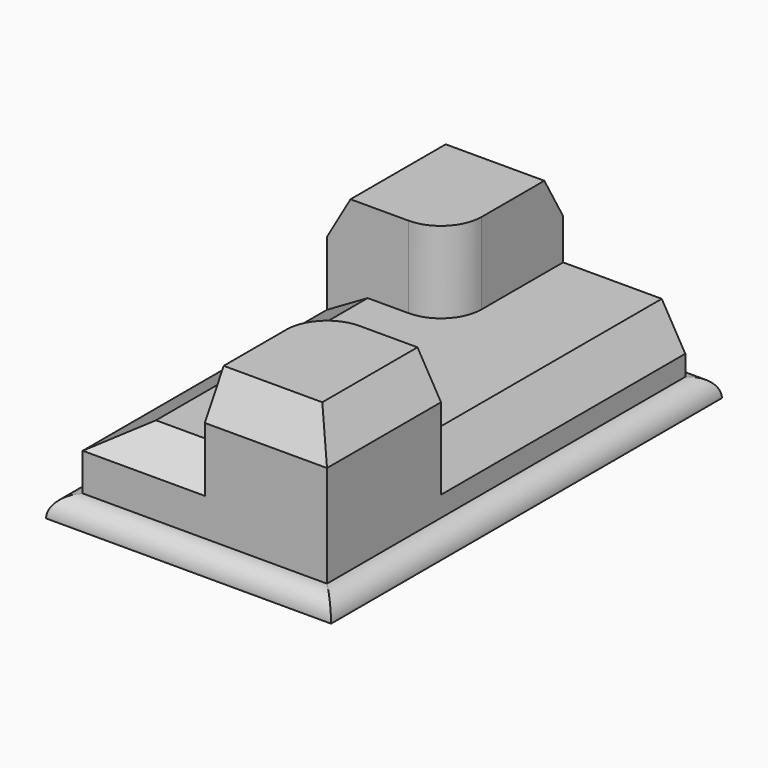
from build123d import *

# Parameters (mm, degrees)
F0_W        = 88.9000063658
F0_H        = 152.4
F1_DEPTH    = 6.35
F2_DEPTH    = 25.4
F3_DEPTH    = 50.8
F4_R        = 6.34999
F5_C1_SIZE2 = 12.7
F5_C1_SIZE  = 7.3323484187
F5_C2_SIZE2 = 7.3323484187
F5_C2_SIZE  = 12.7
F5_C3_SIZE2 = 7.3323484187
F5_C3_SIZE  = 12.7
F5_C4_SIZE2 = 7.3323484187
F5_C4_SIZE  = 12.7
F5_C5_SIZE2 = 12.7
F5_C5_SIZE  = 7.3323484187
F5_C6_SIZE2 = 7.3323484187
F5_C6_SIZE  = 12.7
F6_SIZE2    = 7.3323484187
F6_SIZE     = 12.7


# Not quite as in the source:
# - a fillet or chamfer is up to 0.001 mm smaller than in the source, because OpenCascade refuses the exact size


with BuildPart() as f1:
    # F0 (on Top) → F1 (new body)
    with BuildSketch(Plane.XY):
        with Locations((-12.7734099567, -1.7824335903)):
            Rectangle(F0_W, F0_H)
        Polygon((-50.8734099567, 23.6175632268), (-50.8734099567, 68.0675632268), (-12.7734099567, 68.0675632268), (25.3265900433, 68.0675632268), (25.3265900433, -27.1824304074), (25.3265900433, -71.6324304074), (-12.7734099567, -71.6324304074), (-50.8734099567, -71.6324304074), align=None, mode=Mode.SUBTRACT)
    extrude(amount=F1_DEPTH)

    # F0 (on Top) → F2 (join)
    with BuildSketch(Plane.XY):
        with BuildLine():
            Line((25.3265900433, 68.0675632268), (-12.7734099567, 68.0675632268))
            Line((-12.7734099567, 68.0675632268), (-12.7734099567, 36.3175632268))
            ThreePointArc((-12.7734099567, 36.3175632268), (-16.4931538356, 27.3373071057), (-25.4734099567, 23.6175632268))
            Line((-25.4734099567, 23.6175632268), (-50.8734099567, 23.6175632268))
            Line((-50.8734099567, 23.6175632268), (-50.8734099567, -71.6324304074))
            Line((-50.8734099567, -71.6324304074), (-12.7734099567, -71.6324304074))
            Line((-12.7734099567, -71.6324304074), (-12.7734099567, -39.8824304074))
            ThreePointArc((-12.7734099567, -39.8824304074), (-9.0536660778, -30.9021742863), (-0.0734099567, -27.1824304074))
            Line((-0.0734099567, -27.1824304074), (25.3265900433, -27.1824304074))
            Line((25.3265900433, -27.1824304074), (25.3265900433, 68.0675632268))
        make_face()
    extrude(amount=F2_DEPTH)

    # F0 (on Top) → F3 (join)
    with BuildSketch(Plane.XY):
        with BuildLine():
            Line((-12.7734099567, 68.0675632268), (-50.8734099567, 68.0675632268))
            Line((-50.8734099567, 68.0675632268), (-50.8734099567, 23.6175632268))
            Line((-50.8734099567, 23.6175632268), (-25.4734099567, 23.6175632268))
            ThreePointArc((-25.4734099567, 23.6175632268), (-16.4931538356, 27.3373071057), (-12.7734099567, 36.3175632268))
            Line((-12.7734099567, 36.3175632268), (-12.7734099567, 68.0675632268))
        make_face()
        with BuildLine():
            Line((25.3265900433, -71.6324304074), (25.3265900433, -27.1824304074))
            Line((25.3265900433, -27.1824304074), (-0.0734099567, -27.1824304074))
            ThreePointArc((-0.0734099567, -27.1824304074), (-9.0536660778, -30.9021742863), (-12.7734099567, -39.8824304074))
            Line((-12.7734099567, -39.8824304074), (-12.7734099567, -71.6324304074))
            Line((-12.7734099567, -71.6324304074), (25.3265900433, -71.6324304074))
        make_face()
    extrude(amount=F3_DEPTH)

    # F4 (radius 6.35 in the source; OpenCascade refuses exactly that, so slightly less here)
    f4_edges = [f1.edges().sort_by_distance(p)[0] for p in [
        (31.676593, -1.782434, 6.35),
        (-12.77341, -77.982434, 6.35),
        (-57.223413, -1.782434, 6.35),
        (-12.77341, 74.417566, 6.35),
    ]]
    fillet(f4_edges, radius=F4_R)

    # F5: chamfer of 12.7 x 7.3323484187 on 6 edges, made by hand

    # F5_c1
    f5_c1_edges = [f1.edges().sort_by_distance(p)[0] for p in [
        (-50.8734099567, -24.0074335903, 25.4),
    ]]
    f5_c1_side = f1.faces().sort_by_distance((-50.8734099567, -24.0074335903, 25.2533530316))[0]
    chamfer(f5_c1_edges, length=F5_C1_SIZE, length2=F5_C1_SIZE2, reference=f5_c1_side)

    # F5_c2
    f5_c2_edges = [f1.edges().sort_by_distance(p)[0] for p in [
        (-31.8234099567, 68.0675632268, 50.8),
    ]]
    f5_c2_side = f1.faces().sort_by_distance((-31.8234099567, 68.0675632268, 50.6533530316))[0]
    chamfer(f5_c2_edges, length=F5_C2_SIZE, length2=F5_C2_SIZE2, reference=f5_c2_side)

    # F5_c3
    f5_c3_edges = [f1.edges().sort_by_distance(p)[0] for p in [
        (25.3265900433, -49.4074304074, 50.8),
    ]]
    f5_c3_side = f1.faces().sort_by_distance((25.3265900433, -49.4074304074, 50.6533530316))[0]
    chamfer(f5_c3_edges, length=F5_C3_SIZE, length2=F5_C3_SIZE2, reference=f5_c3_side)

    # F5_c4
    f5_c4_edges = [f1.edges().sort_by_distance(p)[0] for p in [
        (25.3265900433, 20.4425664097, 25.4),
    ]]
    f5_c4_side = f1.faces().sort_by_distance((25.3265900433, 20.4425664097, 25.2533530316))[0]
    chamfer(f5_c4_edges, length=F5_C4_SIZE, length2=F5_C4_SIZE2, reference=f5_c4_side)

    # F5_c5
    f5_c5_edges = [f1.edges().sort_by_distance(p)[0] for p in [
        (-25.4734099567, -71.6324304074, 25.4),
    ]]
    f5_c5_side = f1.faces().sort_by_distance((-25.4734099567, -71.6324304074, 25.2533530316))[0]
    chamfer(f5_c5_edges, length=F5_C5_SIZE, length2=F5_C5_SIZE2, reference=f5_c5_side)

    # F5_c6
    f5_c6_edges = [f1.edges().sort_by_distance(p)[0] for p in [
        (2.610415834, -71.6324304074, 50.8),
    ]]
    f5_c6_side = f1.faces().sort_by_distance((2.610415834, -71.6324304074, 50.6533530316))[0]
    chamfer(f5_c6_edges, length=F5_C6_SIZE, length2=F5_C6_SIZE2, reference=f5_c6_side)

    # F6
    f6_edges = [f1.edges().sort_by_distance(p)[0] for p in [
        (-50.87341, 42.176389, 50.8),
    ]]
    f6_side = f1.faces().sort_by_distance((-50.87341, 66.601552, 22.225))[0]
    chamfer(f6_edges, length=F6_SIZE, length2=F6_SIZE2, reference=f6_side)


solid = f1.part
